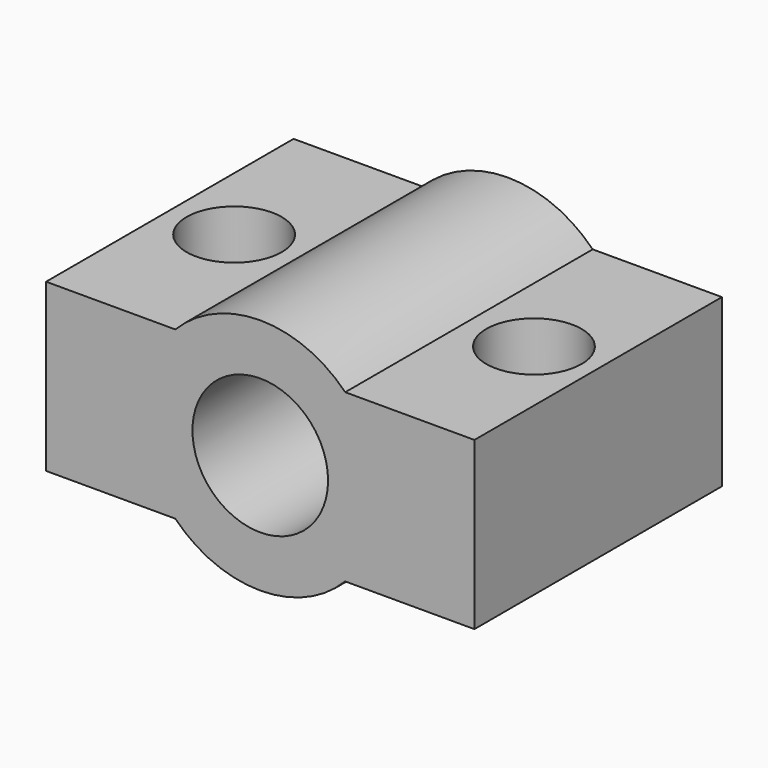
from build123d import *

# Parameters (mm, degrees)
F0_R     = 2.85
F1_DEPTH = 13
F2_R     = 2
F3_DEPTH = 12.5
F4_R     = 2
F5_DEPTH = 12.5


# Not quite as in the source:
# - a feature names something its author has since deleted; it is built from what else it names


with BuildPart() as f1:
    # F0 (on Front) → F1 (new body)
    with BuildSketch(Plane.XZ):
        with BuildLine():
            ThreePointArc((3.5707142143, -3.5), (4.6289075964, -1.8902948088), (5, 0))
            ThreePointArc((5, 0), (4.6289075964, 1.8902948088), (3.5707142143, 3.5))
            Line((3.5707142143, 3.5), (-3.5707142143, 3.5))
            ThreePointArc((-3.5707142143, 3.5), (-5, 0), (-3.5707142143, -3.5))
            Line((-3.5707142143, -3.5), (3.5707142143, -3.5))
        make_face()
        Circle(F0_R, mode=Mode.SUBTRACT)
        with BuildLine():
            ThreePointArc((3.5707142143, 3.5), (4.6289075964, 1.8902948088), (5, 0))
            ThreePointArc((5, 0), (4.6289075964, -1.8902948088), (3.5707142143, -3.5))
            Line((3.5707142143, -3.5), (9, -3.5))
            Line((9, -3.5), (9, 3.5))
            Line((9, 3.5), (3.5707142143, 3.5))
        make_face()
        with BuildLine():
            Line((-3.5707142143, 3.5), (3.5707142143, 3.5))
            ThreePointArc((3.5707142143, 3.5), (0, 5), (-3.5707142143, 3.5))
        make_face()
        with BuildLine():
            ThreePointArc((-3.5707142143, -3.5), (0, -5), (3.5707142143, -3.5))
            Line((3.5707142143, -3.5), (-3.5707142143, -3.5))
        make_face()
        with BuildLine():
            ThreePointArc((-3.5707142143, -3.5), (-5, 0), (-3.5707142143, 3.5))
            Line((-3.5707142143, 3.5), (-9, 3.5))
            Line((-9, 3.5), (-9, -3.5))
            Line((-9, -3.5), (-3.5707142143, -3.5))
        make_face()
    extrude(amount=F1_DEPTH)

    # F2 (on Top) → F3 (cut, symmetric)
    with BuildSketch(Plane.XY):
        with Locations((6.3759502955, -6.5950173885)):
            Circle(F2_R)
    extrude(amount=F3_DEPTH, both=True, mode=Mode.SUBTRACT)

    # F4 (on Top) → F5 (cut, symmetric)
    with BuildSketch(Plane.XY):
        with Locations((-6.2739360146, -6.5290778875)):
            Circle(F4_R)
    extrude(amount=F5_DEPTH, both=True, mode=Mode.SUBTRACT)


solid = f1.part
